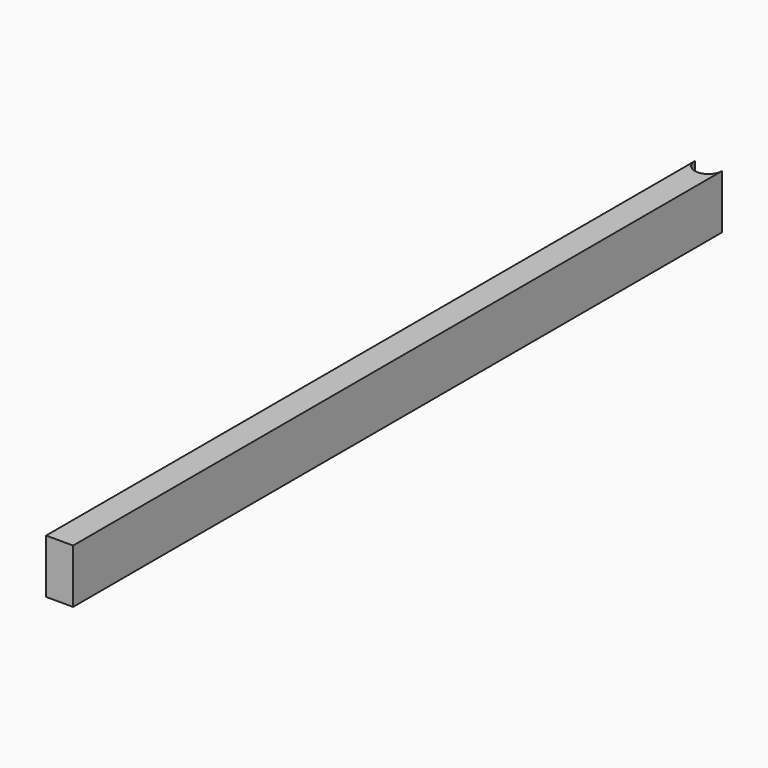
from build123d import *

# Parameters (mm, degrees)
F0_W     = 10
F0_H     = 20
F1_DEPTH = 150
F3_DEPTH = 311


# Not quite as in the source:
# - an extrude ends at something that could not be found from the text; its depth is read off the source's solid


with BuildPart() as f1:
    # F0 (on Front) → F1 (new body, symmetric)
    with BuildSketch(Plane.XZ):
        Rectangle(F0_W, F0_H)
    extrude(amount=F1_DEPTH, both=True)

    # F2 (on face) → F3 (cut, through all)
    with BuildSketch(Plane.XY.offset(10)):
        with BuildLine():
            Line((-5, 150), (5, 150))
            ThreePointArc((5, 150), (0, 155), (-5, 150))
        make_face()
        with BuildLine():
            ThreePointArc((-5, 150), (0, 145), (5, 150))
            Line((5, 150), (-5, 150))
        make_face()
    extrude(amount=-F3_DEPTH, mode=Mode.SUBTRACT)


solid = f1.part
